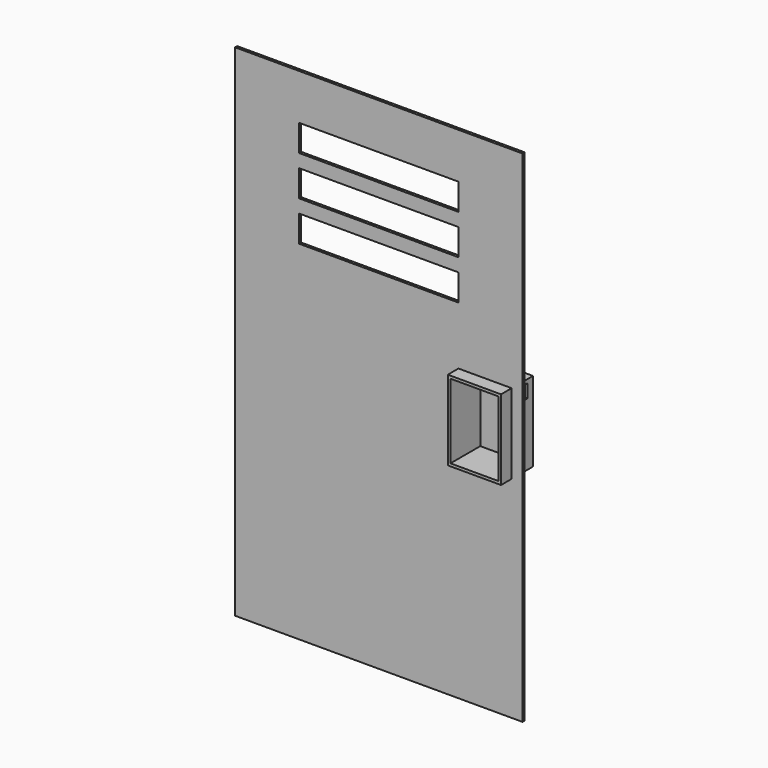
from build123d import *

# Parameters (mm, degrees)
F0_W          = 274.32
F0_H          = 477.52
F1_DEPTH      = 2.54
F2_W          = 152.4
F2_H          = 25.4
F3_W          = 152.4
F3_H          = 25.4
F4_W          = 152.4
F4_H          = 25.4
F5_DEPTH      = 25.4
F6_W          = 45.72
F6_H          = 76.2
F7_DEPTH      = 25.4
F8_W          = 50.8
F8_H          = 76.2
F9_DEPTH      = 12.7
F9_DEPTH_BACK = 25.4
F10_T         = 2.54
F10_T3_DEPTH  = 7.4696609569
F10_T5_DEPTH  = 81.28
F10_T7_DEPTH  = 55.88
F10_T9_DEPTH  = 7.7703390431
F10_T11_DEPTH = 7.62
F11_W         = 13.208
F11_H         = 12.7
F12_DEPTH     = 25.4


# Not quite as in the source:
# - a shell that OpenCascade refuses in one call is made with other operations: the cavity is built on its own and cut out


with BuildPart() as f1:
    # F0 (on Front) → F1 (new body)
    with BuildSketch(Plane.XZ):
        Rectangle(F0_W, F0_H)
    extrude(amount=F1_DEPTH)

    # F2 (on face) + F3 (on face) + F4 (on face) → F5 (cut)
    with BuildSketch(Plane.XZ.offset(2.54)):
        with Locations((0, 182.5210501183)):
            Rectangle(F2_W, F2_H)
    with BuildSketch(Plane.XZ.offset(2.54)):
        with Locations((0, 144.4210501183)):
            Rectangle(F3_W, F3_H)
    with BuildSketch(Plane.XZ.offset(2.54)):
        with Locations((0, 106.3210501183)):
            Rectangle(F4_W, F4_H)
    extrude(amount=-F5_DEPTH, mode=Mode.SUBTRACT)

    # F6 (on face) → F7 (cut)
    with BuildSketch(Plane.XZ.offset(2.54)):
        with Locations((101.6, 0)):
            Rectangle(F6_W, F6_H)
    extrude(amount=-F7_DEPTH, mode=Mode.SUBTRACT)

    # F8 (on face) → F9 (join, two sides)
    with BuildSketch(Plane.XZ.offset(2.54)) as f9_sk:
        with Locations((101.4496609569, 0.1478558406)):
            Rectangle(F8_W, F8_H)
    extrude(amount=F9_DEPTH)
    extrude(f9_sk.sketch, amount=-F9_DEPTH_BACK)

    # F10: shell of thickness 2.54, made by hand


with BuildPart() as f10_core1:
    # F10_t2: copy of F1
    add(f1.part)

    # the walls: a layer under each face that stays
    f10_faces = [f10_core1.faces().sort_by_distance(p)[0] for p in [
        (0, -1.27, 238.76),
        (137.16, -1.27, 0),
        (-137.16, -1.27, 0),
        (0, 0, 0),
        (0, -2.54, 0),
        (0, -1.27, -238.76),
        (101.6, -1.27, -38.1),
        (124.46, -1.27, -38.0260720797),
        (101.4496609569, 3.81, -37.9521441594),
        (126.8496609569, 11.43, 0.1478558406),
        (101.4496609569, 11.43, 38.2478558406),
        (76.0496609569, 11.43, 0.1478558406),
        (78.74, -1.27, -38.0260720797),
        (-76.2, -1.27, 106.3210501183),
        (0, -1.27, 119.0210501183),
        (0, -1.27, 93.6210501183),
        (76.2, -1.27, 106.3210501183),
        (0, -1.27, 131.7210501183),
        (-76.2, -1.27, 144.4210501183),
        (76.2, -1.27, 144.4210501183),
        (0, -1.27, 157.1210501183),
        (0, -1.27, 169.8210501183),
        (-76.2, -1.27, 182.5210501183),
        (76.2, -1.27, 182.5210501183),
        (0, -1.27, 195.2210501183),
        (126.8496609569, -8.89, 0.1478558406),
        (101.4496609569, -8.89, 38.2478558406),
        (76.0496609569, -8.89, 0.1478558406),
        (101.4496609569, 22.86, 0.1478558406),
    ]]
    thicken(f10_faces, amount=-F10_T, mode=Mode.SUBTRACT)

    # F10_s4 → F10_t3 (cut)
    with BuildSketch(Plane.YZ.offset(121.92)):
        Polygon((0.0254, -37.9775441594), (-2.54, -37.9521441594), (-2.54, -35.4121441594), (0, -35.4121441594), align=None)
        Polygon((-2.5654, -37.9775441594), (0, -37.9521441594), (0, -35.4121441594), (-2.54, -35.4121441594), align=None)
    extrude(amount=F10_T3_DEPTH, mode=Mode.SUBTRACT)

    # F10_s6 → F10_t5 (cut)
    with BuildSketch(Plane.XY.offset(-40.4921441594)):
        Polygon((126.8750609569, 0.0254), (126.8496609569, -2.54), (124.3096609569, -2.54), (124.3096609569, 0), align=None)
        Polygon((76.0242609569, 0.0254), (76.0496609569, -2.54), (78.5896609569, -2.54), (78.5896609569, 0), align=None)
        Polygon((126.8750609569, -2.5654), (126.8496609569, 0), (124.3096609569, 0), (124.3096609569, -2.54), align=None)
        Polygon((76.0242609569, -2.5654), (76.0496609569, 0), (78.5896609569, 0), (78.5896609569, -2.54), align=None)
    extrude(amount=F10_T5_DEPTH, mode=Mode.SUBTRACT)

    # F10_s8 → F10_t7 (cut)
    with BuildSketch(Plane.YZ.offset(73.5096609569)):
        Polygon((0.0254, 38.2732558406), (-2.54, 38.2478558406), (-2.54, 35.7078558406), (0, 35.7078558406), align=None)
        Polygon((-2.5654, 38.2732558406), (0, 38.2478558406), (0, 35.7078558406), (-2.54, 35.7078558406), align=None)
    extrude(amount=F10_T7_DEPTH, mode=Mode.SUBTRACT)

    # F10_s10 → F10_t9 (cut)
    with BuildSketch(Plane.YZ.offset(73.5096609569)):
        Polygon((0.0254, -37.9775441594), (-2.54, -37.9521441594), (-2.54, -35.4121441594), (0, -35.4121441594), align=None)
        Polygon((-2.5654, -37.9775441594), (0, -37.9521441594), (0, -35.4121441594), (-2.54, -35.4121441594), align=None)
    extrude(amount=F10_T9_DEPTH, mode=Mode.SUBTRACT)

    # F10_s12 → F10_t11 (cut)
    with BuildSketch(Plane.XZ.offset(-2.54)):
        Polygon((124.4346, -38.0746), (124.46, -40.64), (127, -40.64), (127, -38.1), align=None)
        Polygon((78.7654, -38.0746), (78.74, -40.64), (76.2, -40.64), (76.2, -38.1), align=None)
        Polygon((124.4346, -37.9775441594), (127, -37.9521441594), (127, -35.4121441594), (124.46, -35.4121441594), align=None)
        Polygon((78.7654, -37.9775441594), (78.74, -35.4121441594), (76.2, -35.4121441594), (76.2, -37.9521441594), align=None)
        Polygon((-76.1746, 93.6464501183), (-78.74, 93.6210501183), (-78.74, 91.0810501183), (-76.2, 91.0810501183), align=None)
        Polygon((-76.1746, 118.9956501183), (-78.74, 119.0210501183), (-78.74, 121.5610501183), (-76.2, 121.5610501183), align=None)
        Polygon((76.1746, 118.9956501183), (76.2, 121.5610501183), (78.74, 121.5610501183), (78.74, 119.0210501183), align=None)
        Polygon((76.1746, 93.6464501183), (76.2, 91.0810501183), (78.74, 91.0810501183), (78.74, 93.6210501183), align=None)
        Polygon((76.1746, 131.7464501183), (76.2, 129.1810501183), (78.74, 129.1810501183), (78.74, 131.7210501183), align=None)
        Polygon((-76.1746, 131.7464501183), (-76.2, 129.1810501183), (-78.74, 129.1810501183), (-78.74, 131.7210501183), align=None)
        Polygon((-76.1746, 157.0956501183), (-78.74, 157.1210501183), (-78.74, 159.6610501183), (-76.2, 159.6610501183), align=None)
        Polygon((76.1746, 157.0956501183), (78.74, 157.1210501183), (78.74, 159.6610501183), (76.2, 159.6610501183), align=None)
        Polygon((76.1746, 169.8464501183), (76.2, 167.2810501183), (78.74, 167.2810501183), (78.74, 169.8210501183), align=None)
        Polygon((-76.1746, 169.8464501183), (-76.2, 167.2810501183), (-78.74, 167.2810501183), (-78.74, 169.8210501183), align=None)
        Polygon((-76.1746, 195.1956501183), (-78.74, 195.2210501183), (-78.74, 197.7610501183), (-76.2, 197.7610501183), align=None)
        Polygon((76.1746, 195.1956501183), (78.74, 195.2210501183), (78.74, 197.7610501183), (76.2, 197.7610501183), align=None)
    extrude(amount=F10_T11_DEPTH, mode=Mode.SUBTRACT)


with BuildPart() as f1_1:
    add(f1.part)

    # what is left inside the walls is the cavity
    f10_cavity = [f10_core1.part.solids().sort_by_distance(p)[0] for p in [
        (101.449661, -15.2146, -11.705477),
    ]]
    add(f10_cavity, mode=Mode.SUBTRACT)

    # F11 (on face) → F12 (cut)
    with BuildSketch(Plane.YZ.offset(126.8496609569)):
        with Locations((9.7576510161, 28.402006929)):
            Rectangle(F11_W, F11_H)
    extrude(amount=-F12_DEPTH, mode=Mode.SUBTRACT)


solid = f1_1.part
